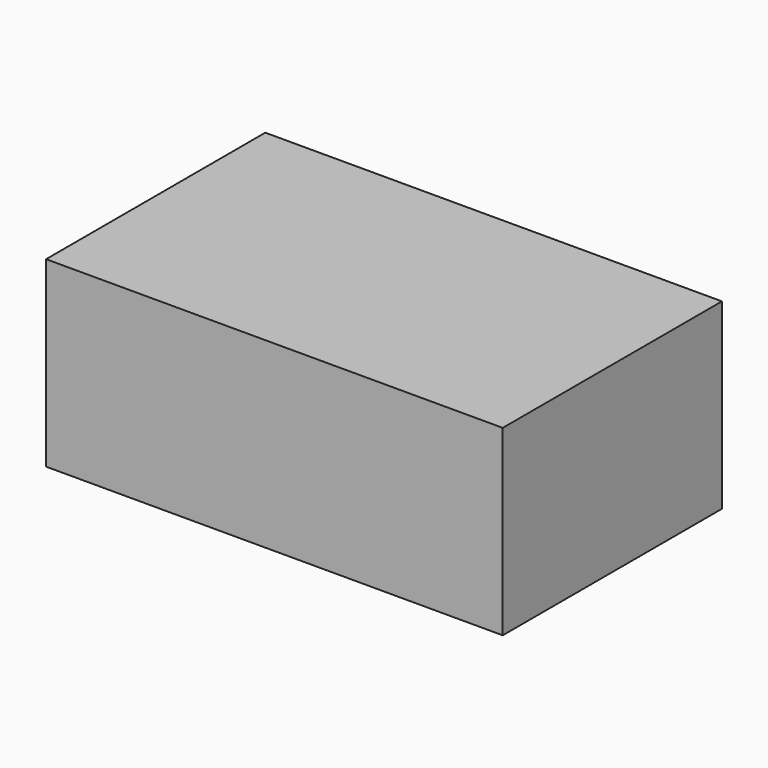
from build123d import *

# Parameters (mm, degrees)
F0_W     = 63.5
F0_H     = 38.1
F1_DEPTH = 25.4


# Not quite as in the source:
# - the program builds the solid bodies; features that only make, move or delete a surface that nothing else refers to are left out


with BuildPart() as f1:
    # F0 (on Top) → F1 (new body)
    with BuildSketch(Plane.XY):
        with Locations((-31.75, 19.05)):
            Rectangle(F0_W, F0_H)
    extrude(amount=F1_DEPTH)


solid = f1.part
